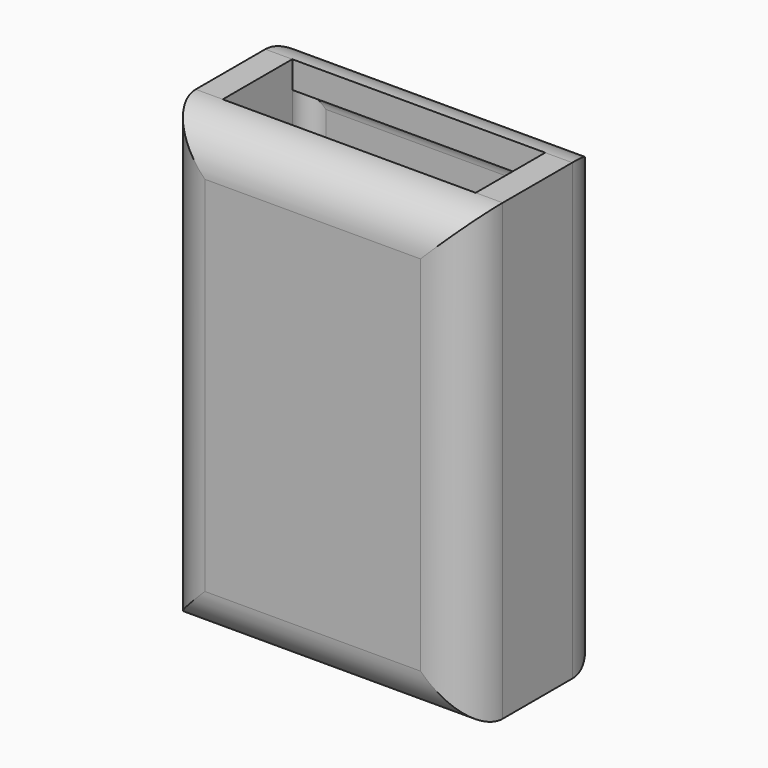
from build123d import *

# Parameters (mm, degrees)
F0_W     = 28.842004016
F0_H     = 16.7503710836
F1_DEPTH = 42.672
F2_R     = 4.2924717139
F3_R     = 4.2926
F4_T     = -2.54


# Not quite as in the source:
# - a shell that OpenCascade refuses in one call is made with other operations: the cavity is built on its own and cut out


with BuildPart() as f1:
    # F0 (on Top) → F1 (new body)
    with BuildSketch(Plane.XY):
        Rectangle(F0_W, F0_H)
    extrude(amount=F1_DEPTH)

    # F2
    f2_edges = [f1.edges().sort_by_distance(p)[0] for p in [
        (-14.421002, -8.375186, 21.336),
        (14.421002, -8.375186, 21.336),
        (0, -8.375186, 0),
        (0, -8.375186, 42.672),
    ]]
    fillet(f2_edges, radius=F2_R)

    # F3
    f3_edges = [f1.edges().sort_by_distance(p)[0] for p in [
        (14.421002, 8.375186, 21.336),
        (-14.421002, 8.375186, 21.336),
        (0, 8.375186, 0),
        (0, 8.375186, 42.672),
    ]]
    fillet(f3_edges, radius=F3_R)

    # F4: a shell. OpenCascade refuses it in one call, so the cavity is built on its own and cut out:
    # the body offset inwards by the wall thickness, plus a prism from it out through each open face.
    f4_core = offset(f1.part, amount=F4_T, mode=Mode.PRIVATE)
    f4_exits = [f4_core.faces().sort_by_distance(p)[0] for p in [
        (0, -6.4e-05, 40.132),
    ]]
    add(f4_core, mode=Mode.SUBTRACT)
    extrude(f4_exits, amount=-F4_T, mode=Mode.SUBTRACT)


solid = f1.part
